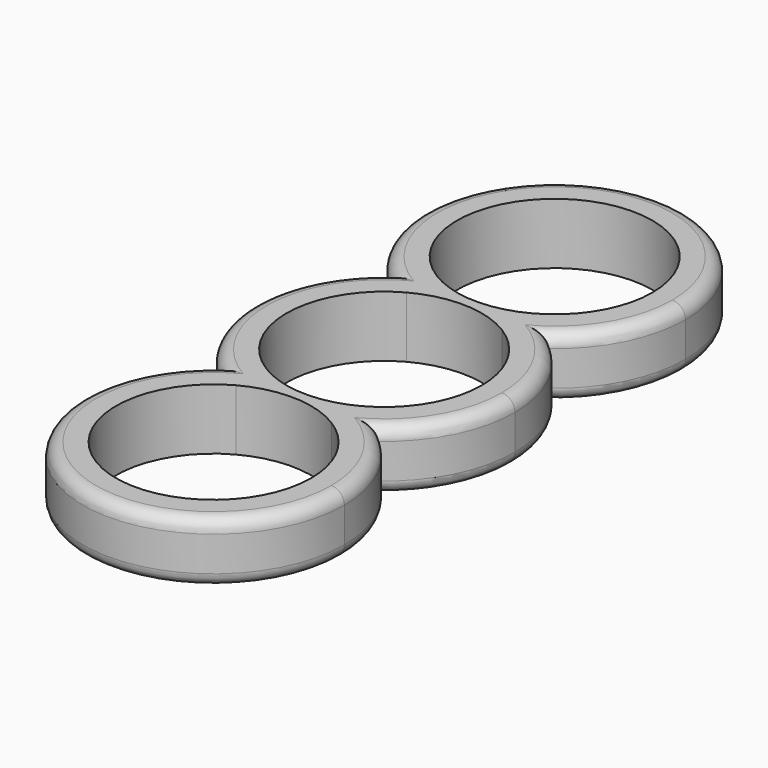
from build123d import *

# Parameters (mm, degrees)
F1_DEPTH = 7
F2_R     = 1.5


# Not quite as in the source:
# - a feature names something its author has since deleted; it is built from what else it names


with BuildPart() as f1:
    # F0 (on Top) → F1 (new body)
    with BuildSketch(Plane.XY):
        with BuildLine():
            ThreePointArc((5.8935462297, 9.5239756845), (9.7838570557, 5.4512513347), (11.2, 0))
            ThreePointArc((11.2, 0), (9.6204369325, -5.734735672), (5.3272869237, -9.8519040816))
            ThreePointArc((5.3272869237, -9.8519040816), (7.197055209, -10.8328912854), (8.9105519184, -12.0667058427))
            ThreePointArc((8.9105519184, -12.0667058427), (13.39151878, -6.7581251296), (15.0001885534, 1.4424e-06))
            ThreePointArc((15.0001885534, 1.4424e-06), (13.5832277592, 6.3640446487), (9.6000490957, 11.5257412263))
            ThreePointArc((9.6000490957, 11.5257412263), (7.8174179542, 10.3940967316), (5.8935462297, 9.5239756845))
        make_face()
        with BuildLine():
            ThreePointArc((-5.3272869237, 9.8519040816), (0.327179857, 11.1952201113), (5.8935462297, 9.5239756845))
            ThreePointArc((5.8935462297, 9.5239756845), (7.8174179542, 10.3940967316), (9.6000490957, 11.5257412263))
            ThreePointArc((9.6000490957, 11.5257412263), (7.8865830002, 12.7594991844), (6.0168567698, 13.7404418856))
            ThreePointArc((6.0168567698, 13.7404418856), (0.3623935251, 12.3970768259), (-5.2039931394, 14.0682811136))
            ThreePointArc((-5.2039931394, 14.0682811136), (-7.1278014357, 13.1981739945), (-8.910376538, 12.066559765))
            ThreePointArc((-8.910376538, 12.066559765), (-7.196958132, 10.832831283), (-5.3272869237, 9.8519040816))
        make_face()
        with BuildLine():
            ThreePointArc((8.9105519184, -12.0667058427), (7.197055209, -10.8328912854), (5.3272869237, -9.8519040816))
            ThreePointArc((5.3272869237, -9.8519040816), (-0.327179857, -11.1952201113), (-5.8935462297, -9.5239756845))
            ThreePointArc((-5.8935462297, -9.5239756845), (-7.8173076322, -10.3940371507), (-9.5998473694, -11.5255922639))
            ThreePointArc((-9.5998473694, -11.5255922639), (-7.8863983485, -12.759377345), (-6.0166850845, -13.740349049))
            ThreePointArc((-6.0166850845, -13.740349049), (-0.3622147698, -12.39708205), (5.2041313094, -14.0683666148))
            ThreePointArc((5.2041313094, -14.0683666148), (7.1279561409, -13.1982912207), (8.9105519184, -12.0667058427))
        make_face()
        with BuildLine():
            ThreePointArc((-5.8935462297, -9.5239756845), (-11.1952201113, 0.327179857), (-5.3272869237, 9.8519040816))
            ThreePointArc((-5.3272869237, 9.8519040816), (-7.196958132, 10.832831283), (-8.910376538, 12.066559765))
            ThreePointArc((-8.910376538, 12.066559765), (-14.9934099745, 0.4381831238), (-9.5998473694, -11.5255922639))
            ThreePointArc((-9.5998473694, -11.5255922639), (-7.8173076322, -10.3940371507), (-5.8935462297, -9.5239756845))
        make_face()
        with BuildLine():
            ThreePointArc((6.0168567698, 13.7404418856), (7.8865830002, 12.7594991844), (9.6000490957, 11.5257412263))
            ThreePointArc((9.6000490957, 11.5257412263), (14.0808707207, 16.8342849133), (15.6894840044, 23.5922995489))
            ThreePointArc((15.6894840044, 23.5922995489), (-5.6745592019, 37.1753387548), (-8.910376538, 12.066559765))
            ThreePointArc((-8.910376538, 12.066559765), (-7.1278014357, 13.1981739945), (-5.2039931394, 14.0682811136))
            ThreePointArc((-5.2039931394, 14.0682811136), (-4.7618028157, 33.3761368332), (11.8894840044, 23.5922995489))
            ThreePointArc((11.8894840044, 23.5922995489), (10.3099459209, 17.8576057895), (6.0168567698, 13.7404418856))
        make_face()
        with BuildLine():
            ThreePointArc((14.3105159956, -23.5922995489), (12.8936036203, -17.228359686), (8.9105519184, -12.0667058427))
            ThreePointArc((8.9105519184, -12.0667058427), (7.1279561409, -13.1982912207), (5.2041313094, -14.0683666148))
            ThreePointArc((5.2041313094, -14.0683666148), (9.0943928222, -18.1410836989), (10.5105159956, -23.5922995489))
            ThreePointArc((10.5105159956, -23.5922995489), (-6.4242615896, -33.2127114969), (-6.0166850845, -13.740349049))
            ThreePointArc((-6.0166850845, -13.740349049), (-7.8863983485, -12.759377345), (-9.5998473694, -11.5255922639))
            ThreePointArc((-9.5998473694, -11.5255922639), (-7.4476105763, -36.9836297755), (14.3105159956, -23.5922995489))
        make_face()
    extrude(amount=F1_DEPTH)

    # F2
    f2_edges = [f1.edges().sort_by_distance(p)[0] for p in [
        (-1.127791, -38.585894, 0),
        (-14.99341, 0.438183, 0),
        (-1.127791, -38.585894, 7),
        (-14.99341, 0.438183, 7),
        (1.127552, 38.585901, 0),
        (1.127552, 38.585901, 7),
        (14.993787, -0.438191, 0),
        (14.993787, -0.438191, 7),
    ]]
    fillet(f2_edges, radius=F2_R)


solid = f1.part
